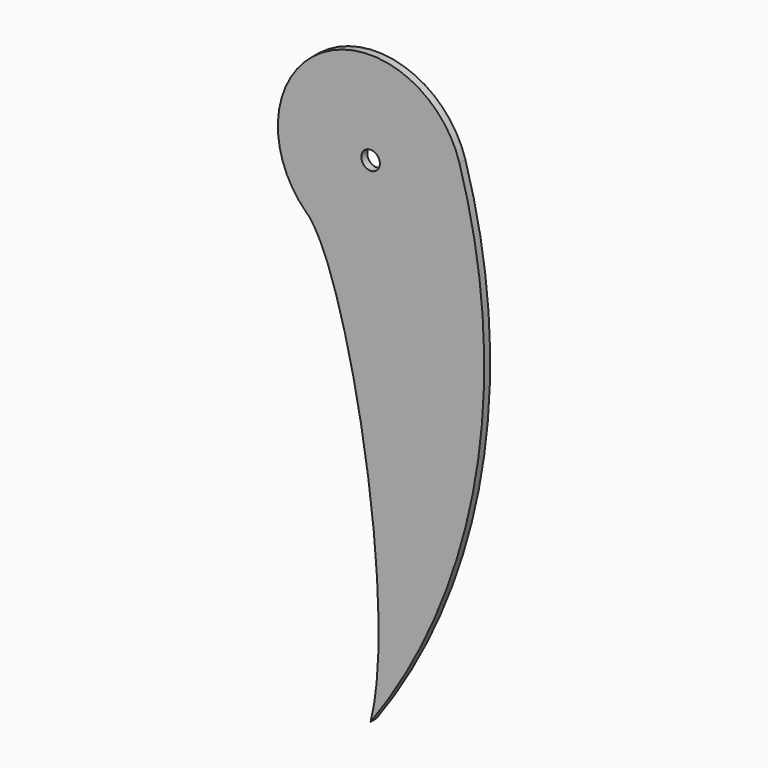
from build123d import *

# Parameters (mm, degrees)
F0_R     = 1.5
F1_DEPTH = 1.2


# Not quite as in the source:
# - a feature names something its author has since deleted; it is built from what else it names


with BuildPart() as f1:
    # F0 (on Front) → F1 (new body)
    with BuildSketch(Plane.XZ):
        with BuildLine():
            ThreePointArc((-10.1224102731, -11.0696346038), (6.0482991784, -13.7265464356), (15, 0))
            ThreePointArc((15, 0), (14.8438679143, 2.1586072693), (14.3787219542, 4.2722774913))
            ThreePointArc((14.3787219542, 4.2722774913), (-7.8146967903, 12.8035352179), (-10.3730753026, -10.8350961587))
            add(Edge.make_bspline(
                [(-10.1224102731, -11.0696346038), (-10.2063109594, -10.9847137567), (-10.2898772286, -10.9064839504), (-10.3730753026, -10.8350961587)],
                knots=[69.0284339282, 69.0284339282, 69.0284339282, 69.0284339282, 69.9384344593, 69.9384344593, 69.9384344593, 69.9384344593], degree=3))
        make_face()
        Circle(F0_R, mode=Mode.SUBTRACT)
        with BuildLine():
            ThreePointArc((14.3787219542, 4.2722774913), (14.8438679143, 2.1586072693), (15, 0))
            ThreePointArc((15, 0), (6.0482991784, -13.7265464356), (-10.1224102731, -11.0696346038))
            add(Edge.make_bspline(
                [(0, -80), (4.5304750858, -62.4535454421), (-3.758092031, -17.5113375297), (-10.1224102731, -11.0696346038)],
                knots=[0, 0, 0, 0, 69.0284339282, 69.0284339282, 69.0284339282, 69.0284339282], degree=3))
            ThreePointArc((0, -80), (17.0066443872, -39.5389078142), (14.3787219542, 4.2722774913))
        make_face()
    extrude(amount=F1_DEPTH)


solid = f1.part
